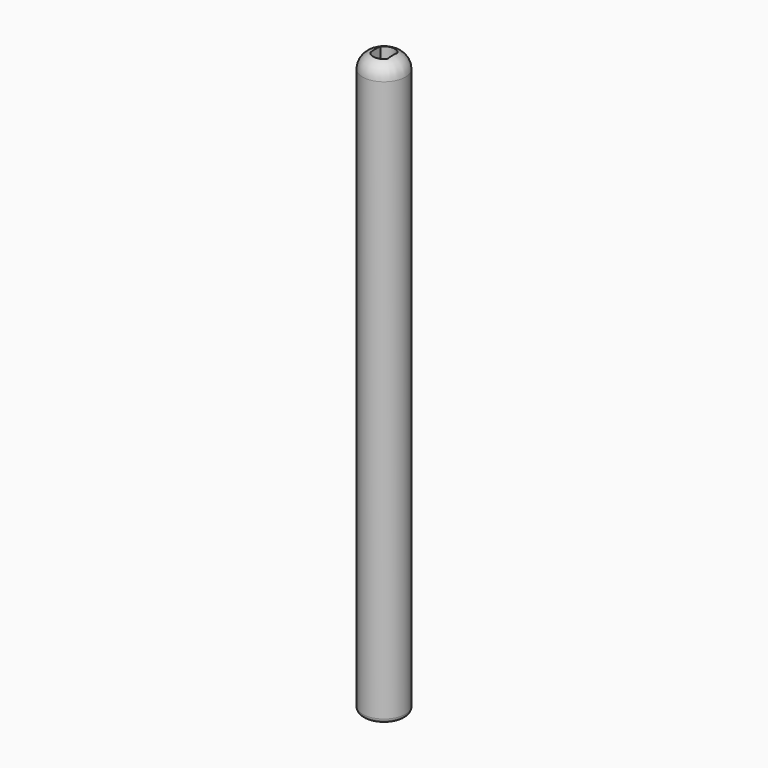
from build123d import *

# Parameters (mm, degrees)
F0_W     = 5
F0_H     = 135
F3_DEPTH = 20
F5_R     = 1


# Not quite as in the source:
# - a fillet or chamfer that OpenCascade refuses, or shapes differently, is made with other operations: its cross-section is extruded or revolved along the edge and cut away or added


with BuildPart() as f1:
    # F0 (on Right) → F1 (revolve)
    with BuildSketch(Plane.YZ):
        with Locations((-2.5, 0)):
            Rectangle(F0_W, F0_H)
    revolve(axis=Axis((0, 0, 0), (0, 0, -1)))

    # F2 (on face) → F3 (cut)
    with BuildSketch(Plane.XY.offset(67.5)):
        with BuildLine():
            Line((-2, 1.5), (-2, -1.5))
            ThreePointArc((-2, -1.5), (0, -2.5), (2, -1.5))
            Line((2, -1.5), (2, 1.5))
            ThreePointArc((2, 1.5), (0, 2.5), (-2, 1.5))
        make_face()
    extrude(amount=-F3_DEPTH, mode=Mode.SUBTRACT)

    # F4: fillet of radius 3.5 on 1 edges, made by hand

    # F4_s1 → F4_t2 (revolve, cut)
    with BuildSketch(Plane.YZ):
        with BuildLine():
            ThreePointArc((-1.5, 67.5), (-3.9748737342, 66.4748737342), (-5, 64))
            Line((-5, 64), (-5, 67.5))
            Line((-5, 67.5), (-1.5, 67.5))
        make_face()
    revolve(axis=Axis((0, 0, 67.5), (0, 0, -1)), mode=Mode.SUBTRACT)

    # F5
    f5_edges = [f1.edges().sort_by_distance(p)[0] for p in [
        (0, 5, -67.5),
    ]]
    fillet(f5_edges, radius=F5_R)


solid = f1.part
